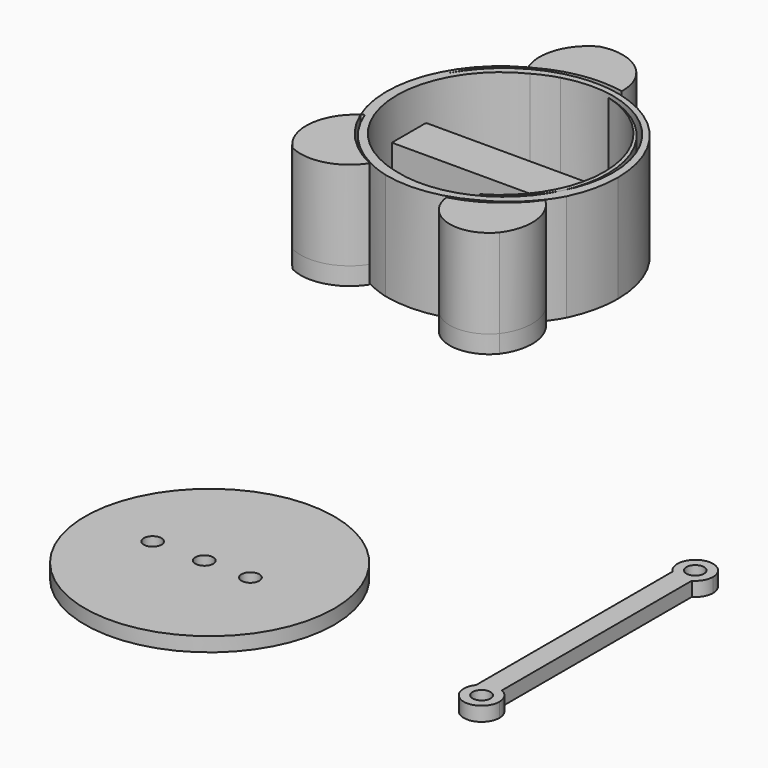
from build123d import *

# Parameters (mm, degrees)
F0_R      = 35
F0_W      = 26.54
F0_H      = 3
F0_R_2    = 1.5
F0_R_3    = 3
F0_W_2    = 26.5384623781
F1_DEPTH  = 4
F2_DEPTH  = 2
F3_D      = 5
F5_DEPTH  = 4
F6_D      = 5
F7_W      = 2
F7_H      = 65
F8_DEPTH  = 3
F10_DEPTH = 30
F11_DEPTH = 5
F12_W     = 42.6740131952
F12_H     = 12
F12_W_2   = 12.3259868048
F13_DEPTH = 20


with BuildPart() as f1:
    # F0 (on Top) → F1 (new body)
    with BuildSketch(Plane.XY):
        with Locations((0, -2.4600220768)):
            Circle(F0_R)
        with Locations((-2.2411635104, -21.1555075496)):
            Rectangle(F0_W, F0_H, mode=Mode.SUBTRACT)
        with Locations((-16, -2.4600220768)):
            Circle(F0_R_2, mode=Mode.SUBTRACT)
        with Locations((-1.5, -2.4600220768)):
            Circle(F0_R_3, mode=Mode.SUBTRACT)
        with Locations((-0.5769231357, 18.5192308724)):
            Rectangle(F0_W_2, F0_H, mode=Mode.SUBTRACT)
        with Locations((11.4414943382, -2.4600220768)):
            Circle(F0_R_2, mode=Mode.SUBTRACT)
        with Locations((-2.2411635104, -21.1555075496)):
            Rectangle(F0_W, F0_H)
        with Locations((-0.5769231357, 18.5192308724)):
            Rectangle(F0_W_2, F0_H)
        with Locations((-1.5, -2.4600220768)):
            Circle(F0_R_3)
        with Locations((11.4414943382, -2.4600220768)):
            Circle(F0_R_2)
        with Locations((-16, -2.4600220768)):
            Circle(F0_R_2)
    extrude(amount=F1_DEPTH)

    # F0 (on Top) → F2 (join)
    with BuildSketch(Plane.XY):
        with Locations((-2.2411635104, -21.1555075496)):
            Rectangle(F0_W, F0_H)
        with Locations((-0.5769231357, 18.5192308724)):
            Rectangle(F0_W_2, F0_H)
    extrude(amount=-F2_DEPTH)

    # F3 (through all)
    with Locations(Plane(origin=(0, 0, 0), x_dir=(1, 0, 0), z_dir=(0, 0, -1))):
        with Locations((-1.5, 2.4600220768), (11.4414943382, 2.4600220768), (-16, 2.4600220768)):
            Hole(F3_D / 2)


with BuildPart() as f5:
    # F4 (on Top) → F5 (new body)
    with BuildSketch(Plane.XY):
        with BuildLine():
            ThreePointArc((87.9450732429, 56.7952425036), (89.7808805629, 58.6259806462), (90.4530596292, 61.1299706553))
            ThreePointArc((90.4530596292, 61.1299706553), (83.5217300265, 65.7419079885), (81.9450732429, 57.5671022163))
            Line((81.9450732429, 57.5671022163), (87.9450732429, 57.5671022163))
            Line((87.9450732429, 57.5671022163), (87.9450732429, 56.7952425036))
        make_face()
        with BuildLine():
            Line((81.9450732429, -12.4328977837), (81.9450732429, -11.3774370589))
            ThreePointArc((81.9450732429, -11.3774370589), (84.3064843691, -19.1548178593), (90.9128758311, -14.4198937342))
            ThreePointArc((90.9128758311, -14.4198937342), (90.105785743, -11.6960166315), (87.9450732429, -9.8515052131))
            Line((87.9450732429, -9.8515052131), (87.9450732429, -12.4328977837))
            Line((87.9450732429, -12.4328977837), (81.9450732429, -12.4328977837))
        make_face()
        with BuildLine():
            ThreePointArc((87.9450732429, 56.7952425036), (84.8151003651, 56.1708368622), (81.9450732429, 57.5671022163))
            Line((81.9450732429, 57.5671022163), (81.9450732429, -11.3774370589))
            ThreePointArc((81.9450732429, -11.3774370589), (84.6804964864, -9.5741490906), (87.9450732429, -9.8515052131))
            Line((87.9450732429, -9.8515052131), (87.9450732429, 56.7952425036))
        make_face()
        with BuildLine():
            Line((87.9450732429, 57.5671022163), (81.9450732429, 57.5671022163))
            ThreePointArc((81.9450732429, 57.5671022163), (84.8151003651, 56.1708368622), (87.9450732429, 56.7952425036))
            Line((87.9450732429, 56.7952425036), (87.9450732429, 57.5671022163))
        make_face()
        with BuildLine():
            ThreePointArc((87.9450732429, -9.8515052131), (84.6804964864, -9.5741490906), (81.9450732429, -11.3774370589))
            Line((81.9450732429, -11.3774370589), (81.9450732429, -12.4328977837))
            Line((81.9450732429, -12.4328977837), (87.9450732429, -12.4328977837))
            Line((87.9450732429, -12.4328977837), (87.9450732429, -9.8515052131))
        make_face()
    extrude(amount=F5_DEPTH)

    # F6 (through all)
    with Locations(Plane(origin=(0, 0, 0), x_dir=(1, 0, 0), z_dir=(0, 0, -1))):
        with Locations((85.4530596292, -61.1299706553), (85.9128758311, 14.4198937342)):
            Hole(F6_D / 2)

    # F7 (on Top) → F8 (join)
    with BuildSketch(Plane.XY):
        with Locations((83.2414569196, 23.0664638802)):
            Rectangle(F7_W, F7_H)
    extrude(amount=F8_DEPTH)


with BuildPart() as f10:
    # F9 (on Top) → F10 (new body)
    with BuildSketch(Plane.XY):
        with BuildLine():
            ThreePointArc((-73.2858614672, 172.2622414718), (-77.0227304851, 159.1962191884), (-75.000224512, 145.7576702356))
            ThreePointArc((-75.000224512, 145.7576702356), (-68.9325789571, 135.7881382146), (-59.6934286842, 128.657500548))
            ThreePointArc((-59.6934286842, 128.657500548), (-56.7023361178, 127.3122486294), (-53.5892591718, 126.2802169468))
            ThreePointArc((-53.5892591718, 126.2802169468), (-41.6838663684, 125.7364505743), (-30.4051696922, 129.586783152))
            ThreePointArc((-30.4051696922, 129.586783152), (-67.0534721321, 135.6434181391), (-73.2858614672, 172.2622414718))
        make_face()
        with BuildLine():
            ThreePointArc((-75.7963746055, 145.2431060979), (-75.4026441809, 145.5071103051), (-75.000224512, 145.7576702356))
            ThreePointArc((-75.000224512, 145.7576702356), (-77.0227304851, 159.1962191884), (-73.2858614672, 172.2622414718))
            ThreePointArc((-73.2858614672, 172.2622414718), (-67.8382371628, 180.1976664827), (-60.2772855271, 186.1541411976))
            ThreePointArc((-60.2772855271, 186.1541411976), (-60.7150688845, 185.9355609592), (-61.1494588106, 185.7103122505))
            ThreePointArc((-61.1494588106, 185.7103122505), (-76.291754107, 168.3067007621), (-75.7963746055, 145.2431060979))
        make_face()
        with BuildLine():
            ThreePointArc((-61.1494588106, 185.7103122505), (-60.7150688845, 185.9355609592), (-60.2772855271, 186.1541411976))
            ThreePointArc((-60.2772855271, 186.1541411976), (-53.6710172386, 188.9768439079), (-46.6015343342, 190.2546712658))
            ThreePointArc((-46.6015343342, 190.2546712658), (-42.2911393785, 190.2500726443), (-38.0204665002, 189.6662242149))
            ThreePointArc((-38.0204665002, 189.6662242149), (-43.1839698715, 200.6995796457), (-55.105868423, 203.2025846503))
            ThreePointArc((-55.105868423, 203.2025846503), (-61.5099400927, 195.6250269593), (-61.1494588106, 185.7103122505))
        make_face()
        with BuildLine():
            ThreePointArc((-14.2020561308, 157.4158754629), (-18.5479392037, 141.3146389581), (-30.4051696922, 129.586783152))
            ThreePointArc((-30.4051696922, 129.586783152), (-24.1386129674, 133.6225846899), (-18.9757059518, 138.9986258344))
            ThreePointArc((-18.9757059518, 138.9986258344), (-17.5480549257, 141.0435895186), (-16.2839985307, 143.1935256462))
            ThreePointArc((-16.2839985307, 143.1935256462), (-13.8983179669, 149.9814104366), (-13.0894609094, 157.1307182312))
            ThreePointArc((-13.0894609094, 157.1307182312), (-19.9857709683, 176.9752326204), (-37.7022578684, 188.2663767473))
            ThreePointArc((-37.7022578684, 188.2663767473), (-20.7462754081, 176.806678123), (-14.2020561308, 157.4158754629))
        make_face()
        with BuildLine():
            ThreePointArc((-49.6290874558, 188.807078357), (-63.4291657743, 183.3538993019), (-73.2858614672, 172.2622414718))
            ThreePointArc((-73.2858614672, 172.2622414718), (-67.0534721321, 135.6434181391), (-30.4051696922, 129.586783152))
            ThreePointArc((-30.4051696922, 129.586783152), (-18.5479392037, 141.3146389581), (-14.2020561308, 157.4158754629))
            ThreePointArc((-14.2020561308, 157.4158754629), (-20.7462754081, 176.806678123), (-37.7022578684, 188.2663767473))
            ThreePointArc((-37.7022578684, 188.2663767473), (-43.6402326559, 189.0978847849), (-49.6290874558, 188.807078357))
        make_face()
        with BuildLine():
            ThreePointArc((-58.9358602723, 183.613950101), (-55.8102922922, 185.1601453587), (-52.5223529313, 186.3217604982))
            ThreePointArc((-52.5223529313, 186.3217604982), (-26.9556144077, 181.5924252869), (-15.3515665912, 158.3250488867))
            ThreePointArc((-15.3515665912, 158.3250488867), (-16.2377535984, 151.1947011831), (-18.8423936526, 144.4982068783))
            ThreePointArc((-18.8423936526, 144.4982068783), (-33.0576562429, 130.6029109503), (-52.8762957046, 129.0619796323))
            ThreePointArc((-52.8762957046, 129.0619796323), (-75.1528317805, 154.2000595569), (-58.9358602723, 183.613950101))
        make_face(mode=Mode.SUBTRACT)
    extrude(amount=F10_DEPTH)


with BuildPart() as f10b:
    # F9 (on Top) → F10, piece 2 (new body)
    with BuildSketch(Plane.XY):
        with BuildLine():
            ThreePointArc((-59.8194696617, 128.4578705467), (-69.380698862, 135.3534521794), (-75.7963746055, 145.2431060979))
            ThreePointArc((-75.7963746055, 145.2431060979), (-81.7781403803, 134.8101403643), (-77.488720417, 123.5749647021))
            ThreePointArc((-77.488720417, 123.5749647021), (-67.7219692241, 122.6434333215), (-59.8194696617, 128.4578705467))
        make_face()
    extrude(amount=F10_DEPTH)


with BuildPart() as f10c:
    # F9 (on Top) → F10, piece 3 (new body)
    with BuildSketch(Plane.XY):
        with BuildLine():
            ThreePointArc((-18.8199962523, 138.8573707921), (-26.5830521793, 131.0249174215), (-36.5439675777, 126.292843082))
            ThreePointArc((-36.5439675777, 126.292843082), (-28.6830339005, 117.0150793111), (-17.0605052263, 120.5911114812))
            ThreePointArc((-17.0605052263, 120.5911114812), (-14.4483808733, 130.0605942776), (-18.8199962523, 138.8573707921))
        make_face()
    extrude(amount=F10_DEPTH)


with BuildPart() as f10d:
    # F9 (on Top) → F10, piece 4 (new body)
    with BuildSketch(Plane.XY):
        with BuildLine():
            ThreePointArc((-31.746594947, 132.1269742486), (-24.3220064999, 137.2982067343), (-18.8423936526, 144.4982068783))
            ThreePointArc((-18.8423936526, 144.4982068783), (-16.6902064444, 150.6521976828), (-15.960628412, 157.1307182312))
            ThreePointArc((-15.960628412, 157.1307182312), (-22.2541626931, 175.2149112747), (-38.4152213356, 185.4846140618))
            ThreePointArc((-38.4152213356, 185.4846140618), (-23.0146642001, 175.0463529979), (-17.0732236334, 157.4158754629))
            ThreePointArc((-17.0732236334, 157.4158754629), (-21.0072194558, 142.7970831878), (-31.746594947, 132.1269742486))
        make_face()
    extrude(amount=F10_DEPTH)


with BuildPart() as f11:
    # F9 (on Top) → F11 (new body)
    with BuildSketch(Plane.XY):
        with BuildLine():
            ThreePointArc((-59.8194696617, 128.4578705467), (-69.380698862, 135.3534521794), (-75.7963746055, 145.2431060979))
            ThreePointArc((-75.7963746055, 145.2431060979), (-81.7781403803, 134.8101403643), (-77.488720417, 123.5749647021))
            ThreePointArc((-77.488720417, 123.5749647021), (-67.7219692241, 122.6434333215), (-59.8194696617, 128.4578705467))
        make_face()
    extrude(amount=F11_DEPTH)


with BuildPart() as f11b:
    # F9 (on Top) → F11, piece 2 (new body)
    with BuildSketch(Plane.XY):
        with BuildLine():
            ThreePointArc((-18.8199962523, 138.8573707921), (-26.5830521793, 131.0249174215), (-36.5439675777, 126.292843082))
            ThreePointArc((-36.5439675777, 126.292843082), (-28.6830339005, 117.0150793111), (-17.0605052263, 120.5911114812))
            ThreePointArc((-17.0605052263, 120.5911114812), (-14.4483808733, 130.0605942776), (-18.8199962523, 138.8573707921))
        make_face()
    extrude(amount=F11_DEPTH)


with BuildPart() as f11c:
    # F9 (on Top) → F11, piece 3 (new body)
    with BuildSketch(Plane.XY):
        with BuildLine():
            ThreePointArc((-61.1494588106, 185.7103122505), (-60.7150688845, 185.9355609592), (-60.2772855271, 186.1541411976))
            ThreePointArc((-60.2772855271, 186.1541411976), (-53.6710172386, 188.9768439079), (-46.6015343342, 190.2546712658))
            ThreePointArc((-46.6015343342, 190.2546712658), (-42.2911393785, 190.2500726443), (-38.0204665002, 189.6662242149))
            ThreePointArc((-38.0204665002, 189.6662242149), (-43.1839698715, 200.6995796457), (-55.105868423, 203.2025846503))
            ThreePointArc((-55.105868423, 203.2025846503), (-61.5099400927, 195.6250269593), (-61.1494588106, 185.7103122505))
        make_face()
    extrude(amount=F11_DEPTH)


with BuildPart() as f13:
    # F12 (on Top) → F13 (new body)
    with BuildSketch(Plane.XY):
        with Locations((-40.4553000044, 160.1312771357)):
            Rectangle(F12_W, F12_H)
        with Locations((-67.9553000044, 160.1312771357)):
            Rectangle(F12_W_2, F12_H)
    extrude(amount=F13_DEPTH)


solid = Compound([f1.part, f5.part, f10.part, f10b.part, f10c.part, f10d.part, f11.part, f11b.part, f11c.part, f13.part])
